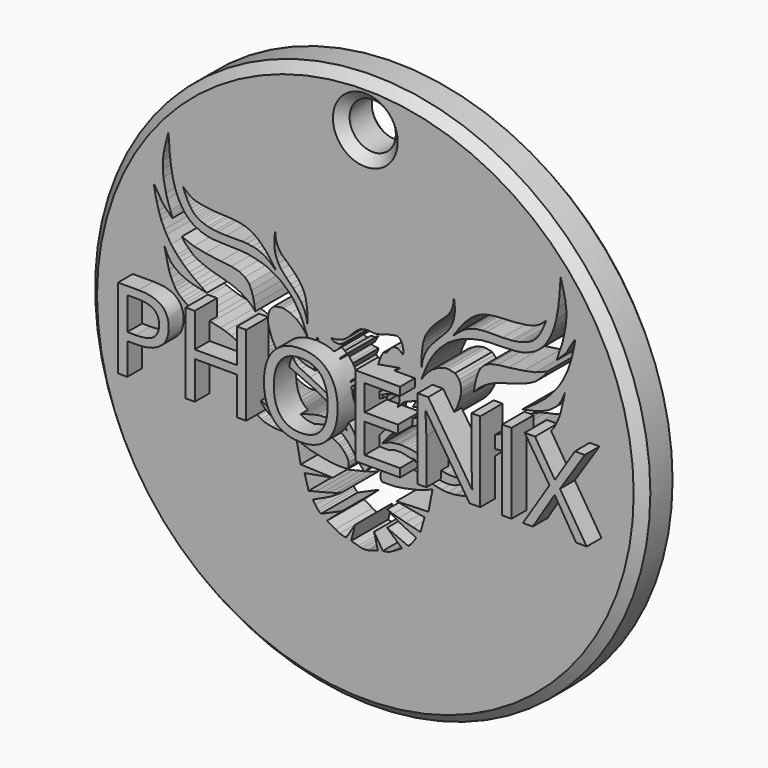
from build123d import *

# Parameters (mm, degrees)
F0_R         = 30
F1_DEPTH     = 5
F3_DEPTH     = 6
F5_START     = 4
F4_TEXT_SIZE = 12.110579539
F5_DEPTH     = 3
F6_R         = 2.5
F7_DEPTH     = 25
F8_SIZE      = 1


# Not quite as in the source:
# - Text() gives the source's letters only with a copy of the font that has no kerning and outlines rounded to 1/6400 em; it was checked with that copy


with BuildPart() as f1:
    # F0 (on Front) → F1 (new body)
    with BuildSketch(Plane.XZ):
        with Locations((-0.3908925251, -0.4964765349)):
            Circle(F0_R)
    extrude(amount=F1_DEPTH)

    # F2 (on Front) → F3 (cut)
    with BuildSketch(Plane.XZ):
        Polygon((-6.9009796716, 3.3349313308), (-6.5914276056, 2.8706034645), (-6.844074931, 3.5021796357), (-7.0858872496, 4.1097938083), (-7.3660952039, 4.7416752204), (-7.6773129404, 5.2794478834), (-7.8633381054, 5.5755167268), (-8.0336434767, 5.8401445858), (-8.2278484479, 6.1087491922), (-8.6159808561, 6.5514193848), (-9.1884760186, 7.0818513632), (-9.5344837755, 7.3751141317), (-10.111220181, 7.7330595814), (-10.5915460736, 7.9969679937), (-11.0050672665, 8.1910705194), (-11.4291384816, 8.3514153957), (-12.170586735, 8.565209806), (-13.1030725315, 8.7572177872), (-13.9272995293, 8.8297724724), (-15.3120374307, 8.863019757), (-16.7676210403, 8.9269923046), (-17.4451787025, 9.0234624222), (-18.1944258511, 9.2512723058), (-18.9065337181, 9.5856180415), (-19.2718468606, 9.8555041477), (-19.5480845869, 10.1086637005), (-19.8738295585, 10.4359621182), (-20.1065801084, 10.7434652746), (-20.4004887491, 11.2334582955), (-20.6413529813, 11.6951130331), (-20.7818560302, 12.0313186198), (-20.96250467, 12.5180631876), (-21.2009325624, 13.3876278996), (-21.4092768729, 14.5726772025), (-21.5388201177, 15.719242394), (-21.5902812779, 16.5217351168), (-21.6488484293, 17.2635931522), (-21.6683708131, 17.5434164703), (-21.8048263341, 17.0381870121), (-21.9664536417, 16.4239984006), (-22.1739932895, 15.4715124518), (-22.2793165594, 14.6293323487), (-22.2793165594, 13.8129889965), (-22.2095865756, 13.0682913586), (-21.9386145473, 11.6732902825), (-21.7981114984, 11.1614549533), (-21.4531756938, 10.173773393), (-21.377377212, 9.9247004837), (-21.3046371937, 9.7339823842), (-21.246092394, 9.5060067251), (-21.4333534241, 9.6954731271), (-21.5672496706, 9.834151715), (-21.839980036, 10.11552196), (-22.0640357584, 10.340699926), (-22.2723558545, 10.5769401416), (-22.3979391158, 10.74438449), (-22.4664080888, 10.8877671883), (-22.6057190448, 11.1188190058), (-22.8970702738, 11.6094984114), (-22.9983050376, 11.7736626416), (-23.1433175504, 12.0034934953), (-23.2253987342, 12.0978886262), (-23.2127886266, 11.8879470974), (-23.1080465019, 11.3241076469), (-22.9371320456, 10.5622867122), (-22.7170959115, 9.7489971668), (-22.5869454443, 9.3390233815), (-22.4437788129, 8.935556747), (-22.0956355333, 8.1833088771), (-21.8711271882, 7.7473041601), (-21.3806033134, 6.9752070121), (-20.7347813994, 6.1996374279), (-20.5585248768, 6.0046529397), (-20.2825926244, 5.7213520631), (-19.9078507721, 5.3766006604), (-19.4278676063, 4.9743568525), (-19.1152207553, 4.7224150039), (-18.7558140606, 4.458708223), (-18.3370038867, 4.1675912216), (-18.016314134, 3.9481716231), (-17.5145696032, 3.6100379748), (-18.3822226251, 3.7996887131), (-18.9730655402, 3.9288345724), (-19.6079221196, 4.1365632488), (-19.850788638, 4.2308908887), (-20.2664192766, 4.4228830375), (-20.6319325281, 4.6325615132), (-20.9945701038, 4.9115952627), (-21.1902355569, 5.0785678585), (-21.430300944, 5.3341447191), (-21.6075535864, 5.6020328775), (-21.7487941244, 5.8274169327), (-21.8645335297, 6.0821418594), (-22.052251676, 6.4952811086), (-22.143593058, 6.7417933606), (-21.8687430024, 5.5104247294), (-21.7532683164, 5.0212959759), (-21.5998519291, 4.4266222568), (-21.3759932667, 3.8224721793), (-21.1102589965, 3.2944113482), (-20.9858700509, 3.0643832629), (-20.816994831, 2.8091561981), (-20.5768158773, 2.5236710225), (-20.2444986021, 2.2400855596), (-19.9949573725, 2.0480745006), (-19.7460502386, 1.8908699276), (-19.3919268787, 1.7100296436), (-18.7242198735, 1.4506969601), (-18.1349273771, 1.265995088), (-17.4961388111, 1.1113942601), (-17.0138068497, 0.9861360304), (-16.0548575222, 0.776529836), (-15.4994018376, 0.6271853927), (-14.9125047028, 0.3992386919), (-14.462351799, 0.1868291292), (-14.191233553, 0.0221533028), (-13.8414734975, -0.2469717583), (-13.7188884659, -0.3515806231), (-13.5706374333, -0.4838758298), (-13.4206879884, -0.6435140385), (-13.1936527732, -0.9473082846), (-13.0392471328, -1.1806669645), (-12.9114612937, -1.4318333706), (-12.7589125186, -1.7675701529), (-12.6668820158, -1.9539315253), (-12.6758497208, -2.0026378334), (-12.9692815244, -1.8056348199), (-13.1037309766, -1.7221844755), (-13.3441239595, -1.5867486363), (-13.5315451771, -1.4814096503), (-13.7764243409, -1.3569180155), (-14.0087269247, -1.2713534525), (-14.3553037196, -1.1796122417), (-14.5744634792, -1.1303438805), (-14.9550195783, -1.0606886353), (-15.3880430592, -1.0301302617), (-15.4070062563, -1.0419205064), (-14.3769606948, -1.9611052703), (-13.950872235, -2.4897714611), (-13.8280401006, -2.6754119899), (-13.7659199536, -2.7864235453), (-13.6367864907, -3.0263995286), (-13.5693699121, -3.1559108756), (-13.4732011494, -3.3553417639), (-13.3834818983, -3.5782567641), (-13.3483398499, -3.665570129), (-13.3177542287, -3.7415626689), (-13.2900051499, -3.8164519222), (-13.2579220653, -3.8961650353), (-13.1716039032, -4.1291206144), (-13.1037309766, -4.2977565899), (-13.0368275568, -4.5038657263), (-12.9336360842, -4.755594302), (-12.8743490204, -4.9155983143), (-12.8289693967, -5.0395550206), (-12.7818249166, -5.179558415), (-12.7129619941, -5.3162728436), (-12.6529606059, -5.441990681), (-12.5875174999, -5.5690663867), (-12.5018004328, -5.717641674), (-12.4399675409, -5.8170924781), (-12.3709030449, -5.8906194754), (-12.2719677165, -6.0149733908), (-12.2122876346, -6.0785096139), (-12.1162394062, -6.1718025245), (-11.9583159685, -6.3006826676), (-11.6442255676, -6.48872694), (-11.4394053817, -6.5820780583), (-11.263766326, -6.651269272), (-10.9468530864, -6.7377560772), (-10.4531301185, -6.8261306733), (-10.1994303986, -6.8651614711), (-9.4673996791, -6.9074714556), (-8.8127674535, -6.8461140618), (-8.1605101004, -6.7201512866), (-7.7530797571, -6.601061672), (-7.6366481371, -6.5667750314), (-7.1542183869, -6.3989814371), (-6.7082373425, -6.2484969385), (-6.3224504702, -6.1034848914), (-6.0155452229, -5.9889322147), (-5.7466630824, -5.8877016418), (-5.4877381772, -5.793986842), (-5.3067770787, -5.7256827131), (-5.0938818604, -5.6618140079), (-4.9314326607, -5.6130257435), (-4.4543091208, -5.6298798881), (-4.2681246996, -5.6629236788), (-3.8872428704, -5.7842899114), (-3.6318132188, -5.9038903564), (-3.3626011573, -6.0657951981), (-3.2329140231, -6.1565763317), (-3.1198710203, -6.2322891317), (-3.0065586325, -6.325469818), (-2.8050330002, -6.5247113816), (-2.6203475427, -6.7271809094), (-2.4301900994, -6.9857402705), (-2.3060552776, -7.2086802684), (-2.1962239407, -7.4997954071), (-2.1979229059, -7.8905448318), (-2.2251054179, -7.9788882285), (-2.2998573259, -8.1215966493), (-2.3934820201, -8.2066971809), (-2.5116000324, -8.2011017948), (-3.1098364852, -8.2135656849), (-3.6893782672, -8.1886388361), (-4.1131288745, -8.13878607), (-4.7487551346, -8.0390796065), (-5.3594545461, -7.9144472256), (-6.4499899745, -7.6651819982), (-7.2787967511, -7.3722954839), (-7.8291641548, -7.1412432007), (-7.3802727275, -9.4111217186), (-3.9100204594, -9.5452908427), (-5.1035000943, -9.7587769851), (-5.6091333916, -9.8464553431), (-6.3824308752, -9.9857078539), (-6.9622276351, -10.0901154801), (-6.5257768147, -11.6362702101), (-5.7188435458, -11.4410445094), (-4.9314326607, -11.2490728498), (-4.1830670089, -11.0505931079), (-3.5453294404, -10.874889791), (-2.9302015544, -10.6291441345), (-3.2655058894, -10.8683817089), (-4.1545955464, -11.4114684984), (-4.7202953137, -11.6943186149), (-5.962850526, -12.2760608792), (-6.0480938971, -12.3117221519), (-6.0583320446, -12.3439328745), (-5.7991264497, -12.7167284), (-5.5476897396, -13.0691304803), (-5.4026274078, -13.2278686718), (-5.2478690632, -13.359698467), (-5.1814815961, -13.3798383176), (-5.1269410178, -13.3649753407), (-2.913645003, -12.3976254836), (-4.5224814676, -13.8263506815), (-3.6250384645, -14.3688376834), (-3.1727361493, -14.6062457934), (-2.6696813293, -14.7449653596), (-2.4519131985, -14.7449653596), (-1.5037892153, -13.2389152423), (-1.9168391591, -14.9040902033), (-1.1345401872, -15.122467652), (-0.889661198, -15.2004463598), (-0.6817192771, -15.2363106608), (-0.4773337569, -15.2363106608), (-0.2729482367, -15.2363106608), (-0.0650063157, -15.2004463598), (0.1798726735, -15.122467652), (0.9621716454, -14.9040902033), (0.5491217016, -13.2389152423), (1.4972456847, -14.7449653596), (1.7150138156, -14.7449653596), (2.2180686356, -14.6062457934), (2.6703709508, -14.3688376834), (3.5678139539, -13.8263506815), (1.9589774893, -12.3976254836), (4.1722735041, -13.3649753407), (4.2268140824, -13.3798383176), (4.2932015494, -13.359698467), (4.4479598941, -13.2278686718), (4.5930222259, -13.0691304803), (4.844458936, -12.7167284), (5.1036645309, -12.3439328745), (5.0934263834, -12.3117221519), (5.0081830123, -12.2760608792), (3.7656278, -11.6943186149), (3.1999280327, -11.4114684984), (2.3108383757, -10.8683817089), (1.9755340406, -10.6291441345), (2.5906619267, -10.874889791), (3.2283994951, -11.0505931079), (3.9767651469, -11.2490728498), (4.764176032, -11.4410445094), (5.5711093009, -11.6362702101), (6.0075601214, -10.0901154801), (5.4277633614, -9.9857078539), (4.6544658779, -9.8464553431), (4.1488325805, -9.7587769851), (2.9553529457, -9.5452908427), (6.4256052137, -9.4111217186), (6.8744966411, -7.1412432007), (6.3241292373, -7.3722954839), (5.4953224608, -7.6651819982), (4.4047870324, -7.9144472256), (3.7940876209, -8.0390796065), (3.1584613607, -8.13878607), (2.7347107534, -8.1886388361), (2.1551689715, -8.2135656849), (1.5569325187, -8.2011017948), (1.4388145064, -8.2066971809), (1.3451898121, -8.1215966493), (1.2704379042, -7.9788882285), (1.2432553922, -7.8905448318), (1.241556427, -7.4997954071), (1.3513877639, -7.2086802684), (1.4755225857, -6.9857402705), (1.665680029, -6.7271809094), (1.8503654865, -6.5247113816), (2.0518911188, -6.325469818), (2.1652035066, -6.2322891317), (2.2782465094, -6.1565763317), (2.4079336436, -6.0657951981), (2.6771457051, -5.9038903564), (2.9325753567, -5.7842899114), (3.3134571859, -5.6629236788), (3.499641607, -5.6298798881), (3.9767651469, -5.6130257435), (4.1392143467, -5.6618140079), (4.3521095649, -5.7256827131), (4.5330706635, -5.793986842), (4.7919955687, -5.8877016418), (5.0608777092, -5.9889322147), (5.3677829565, -6.1034848914), (5.7535698288, -6.2484969385), (6.1995508731, -6.3989814371), (6.6819806234, -6.5667750314), (6.7984122434, -6.601061672), (7.2058425867, -6.7201512866), (7.8580999398, -6.8461140618), (8.5127321654, -6.9074714556), (9.2447628849, -6.8651614711), (9.4984626048, -6.8261306733), (9.9921855726, -6.7377560772), (10.3090988123, -6.651269272), (10.484737868, -6.5820780583), (10.6895580539, -6.48872694), (11.0036484548, -6.3006826676), (11.1615718924, -6.1718025245), (11.2576201209, -6.0785096139), (11.3173002028, -6.0149733908), (11.4162355312, -5.8906194754), (11.4853000272, -5.8170924781), (11.5471329191, -5.717641674), (11.6328499862, -5.5690663867), (11.6982930922, -5.441990681), (11.7582944804, -5.3162728436), (11.8271574029, -5.179558415), (11.8743018829, -5.0395550206), (11.9196815067, -4.9155983143), (11.9789685705, -4.755594302), (12.0821600431, -4.5038657263), (12.1490634629, -4.2977565899), (12.2169363894, -4.1291206144), (12.3032545516, -3.8961650353), (12.3353376362, -3.8164519222), (12.363086715, -3.7415626689), (12.3936723362, -3.665570129), (12.4288143846, -3.5782567641), (12.5185336357, -3.3553417639), (12.6147023984, -3.1559108756), (12.682118977, -3.0263995286), (12.8112524399, -2.7864235453), (12.8733725869, -2.6754119899), (12.9962047213, -2.4897714611), (13.4222931811, -1.9611052703), (14.4523387426, -1.0419205064), (14.4333755455, -1.0301302617), (14.0003520646, -1.0606886353), (13.6197959655, -1.1303438805), (13.4006362059, -1.1796122417), (13.0540594109, -1.2713534525), (12.8217568272, -1.3569180155), (12.5768776634, -1.4814096503), (12.3894564458, -1.5867486363), (12.1490634629, -1.7221844755), (12.0146140107, -1.8056348199), (11.7211822071, -2.0026378334), (11.712214502, -1.9539315253), (11.8042450049, -1.7675701529), (11.95679378, -1.4318333706), (12.0845796191, -1.1806669645), (12.2389852594, -0.9473082846), (12.4660204747, -0.6435140385), (12.6159699196, -0.4838758298), (12.7642209522, -0.3515806231), (12.8868059837, -0.2469717583), (13.2365660393, 0.0221533028), (13.5076842853, 0.1868291292), (13.9578371891, 0.3992386919), (14.5447343239, 0.6271853927), (15.1001900085, 0.776529836), (16.059139336, 0.9861360304), (16.5414712974, 1.1113942601), (17.1802598634, 1.265995088), (17.7695523598, 1.4506969601), (18.437259365, 1.7100296436), (18.7913827249, 1.8908699276), (19.0402898588, 2.0480745006), (19.2898310884, 2.2400855596), (19.6221483636, 2.5236710225), (19.8623273172, 2.8091561981), (20.0312025372, 3.0643832629), (20.1555914828, 3.2944113482), (20.421325753, 3.8224721793), (20.6451844154, 4.4266222568), (20.7986008027, 5.0212959759), (20.9140754887, 5.5104247294), (21.1889255443, 6.7417933606), (21.0975841623, 6.4952811086), (20.909866016, 6.0821418594), (20.7941266106, 5.8274169327), (20.6528860726, 5.6020328775), (20.4756334302, 5.3341447191), (20.2355680432, 5.0785678585), (20.0399025901, 4.9115952627), (19.6772650143, 4.6325615132), (19.3117517629, 4.4228830375), (18.8961211243, 4.2308908887), (18.6532546059, 4.1365632488), (18.0183980265, 3.9288345724), (17.4275551114, 3.7996887131), (16.5599020895, 3.6100379748), (17.0616466203, 3.9481716231), (17.382336373, 4.1675912216), (17.8011465468, 4.458708223), (18.1605532416, 4.7224150039), (18.4732000926, 4.9743568525), (18.9531832584, 5.3766006604), (19.3279251107, 5.7213520631), (19.6038573631, 6.0046529397), (19.7801138856, 6.1996374279), (20.4259357997, 6.9752070121), (20.9164596745, 7.7473041601), (21.1409680196, 8.1833088771), (21.4891112992, 8.935556747), (21.6322779306, 9.3390233815), (21.7624283978, 9.7489971668), (21.9824645319, 10.5622867122), (22.1533789882, 11.3241076469), (22.2581211128, 11.8879470974), (22.2707312205, 12.0978886262), (22.1886500367, 12.0034934953), (22.0436375239, 11.7736626416), (21.94240276, 11.6094984114), (21.6510515311, 11.1188190058), (21.5117405751, 10.8877671883), (21.443271602, 10.74438449), (21.3176883408, 10.5769401416), (21.1093682447, 10.340699926), (20.8853125223, 10.11552196), (20.6125821569, 9.834151715), (20.4786859103, 9.6954731271), (20.2914248803, 9.5060067251), (20.34996968, 9.7339823842), (20.4227096983, 9.9247004837), (20.49850818, 10.173773393), (20.8434439846, 11.1614549533), (20.9839470335, 11.6732902825), (21.2549190619, 13.0682913586), (21.3246490457, 13.8129889965), (21.3246490457, 14.6293323487), (21.2193257757, 15.4715124518), (21.0117861279, 16.4239984006), (20.8501588204, 17.0381870121), (20.7137032994, 17.5434164703), (20.6941809156, 17.2635931522), (20.6356137642, 16.5217351168), (20.584152604, 15.719242394), (20.4546093591, 14.5726772025), (20.2462650486, 13.3876278996), (20.0078371563, 12.5180631876), (19.8271885165, 12.0313186198), (19.6866854676, 11.6951130331), (19.4458212354, 11.2334582955), (19.1519125947, 10.7434652746), (18.9191620448, 10.4359621182), (18.5934170731, 10.1086637005), (18.3171793469, 9.8555041477), (17.9518662044, 9.5856180415), (17.2397583374, 9.2512723058), (16.4905111887, 9.0234624222), (15.8129535266, 8.9269923046), (14.357369917, 8.863019757), (12.9726320156, 8.8297724724), (12.1484050178, 8.7572177872), (11.2159192213, 8.565209806), (10.4744709679, 8.3514153957), (10.0503997528, 8.1910705194), (9.6368785598, 7.9969679937), (9.1565526673, 7.7330595814), (8.5798162618, 7.3751141317), (8.2338085049, 7.0818513632), (7.6613133424, 6.5514193848), (7.2731809341, 6.1087491922), (7.0789759629, 5.8401445858), (6.9086705917, 5.5755167268), (6.7226454266, 5.2794478834), (6.4114276902, 4.7416752204), (6.1312197358, 4.1097938083), (5.8894074173, 3.5021796357), (5.6367600919, 2.8706034645), (5.9463121579, 3.3349313308), (6.3255131827, 3.7837815471), (6.8517514155, 4.2481096461), (7.5172880315, 4.619571846), (8.2911677309, 4.8439968377), (8.6161974468, 4.8439968377), (9.3043926754, 4.6935421415), (9.5365564921, 4.4768559746), (9.7455042996, 4.244692158), (9.8770638579, 3.8887073752), (9.9699288257, 3.4553345758), (9.9699288257, 3.1767380424), (9.8920525634, 2.6312284172), (9.7465864965, 2.1786685102), (9.5263780677, 1.5331205213), (9.2516099685, 1.0320723522), (8.9566377574, 0.5673905252), (8.4863552474, 0.0535830186), (7.900582219, -0.4137892101), (7.1590175503, -0.7752237143), (6.4922334277, -1.0494154412), (5.769364594, -1.3734601671), (5.3143613623, -1.5531850513), (4.8175803968, -1.799066551), (4.4362131157, -1.9797142595), (4.0548458346, -2.1954877302), (3.5897002096, -2.4586620791), (3.1866920763, -2.7417927049), (2.747433784, -3.0866917223), (2.4477891275, -3.3350461163), (2.3023235262, -3.4805119503), (2.1528171492, -3.642140422), (1.975025807, -3.8441759534), (1.8526418717, -3.9994004183), (1.7260537134, -4.1428669356), (1.6142340028, -4.2842240073), (1.5298179933, -4.4043259695), (1.4482704573, -4.5198518783), (1.4057977241, -4.5878081582), (1.4877891984, -4.5414182715), (1.5742309042, -4.4837985188), (1.6762433224, -4.4358973391), (1.7399483764, -4.4059838513), (1.8232696117, -4.3668593453), (1.911158617, -4.3255899871), (2.0272262045, -4.2825178243), (2.1301748347, -4.2452458292), (2.2677017234, -4.1954549626), (2.4408279569, -4.1494057514), (2.5509885163, -4.1262721643), (2.7810983011, -4.0910816751), (3.0116653652, -4.0648807772), (3.1651710742, -4.0402412415), (3.2942542466, -4.0255726458), (3.4481315524, -4.0255726458), (3.672859224, -4.0362342261), (3.9383466938, -4.0648807772), (4.3332051137, -4.0804566815), (4.6627936536, -4.1280263104), (4.8678224557, -4.179386422), (5.1014274941, -4.2290138081), (5.3231935599, -4.2778020725), (5.5955220596, -4.3665086851), (5.8127130033, -4.422603175), (5.9507582919, -4.4709192589), (6.0827513807, -4.5081526041), (6.2150448211, -4.5535927638), (6.3577858573, -4.6026214645), (6.5070544952, -4.6633598395), (6.6908556619, -4.7135576606), (6.8142712698, -4.7468063422), (6.9485898712, -4.7857123427), (7.088004204, -4.8394398764), (7.2577461251, -4.8865387216), (7.5232326635, -4.965854343), (7.8349873074, -5.0506782718), (8.0614272156, -5.0962027162), (8.4007005789, -5.1536601968), (8.6362141354, -5.1790725115), (8.9883797973, -5.1929643228), (9.1500332945, -5.1993410374), (9.3879853957, -5.1885233261), (9.5861627829, -5.1660030866), (9.7404071712, -5.1298472099), (9.8646483966, -5.096486304), (9.9701821455, -5.0710150972), (10.0580757135, -5.0332737155), (10.146530869, -4.9977004528), (10.2327583008, -4.9671088345), (10.32118086, -4.9322033301), (10.3755673044, -4.9044843763), (10.4311477044, -4.8715993762), (10.4972781264, -4.8379208893), (10.5630481266, -4.8027201556), (10.6181647279, -4.773077555), (10.7272188761, -4.7092679888), (10.8612436452, -4.630937241), (10.8412739033, -4.6890766901), (10.7994867139, -4.7463122755), (10.7605807134, -4.8018926755), (10.7114841812, -4.8639569432), (10.6834998748, -4.8993326695), (10.6483479613, -4.940148443), (10.6192342784, -4.9817397171), (10.5811642134, -5.0188680179), (10.5499748524, -5.0582953413), (10.5216738761, -5.0987255978), (10.4824812734, -5.1451963373), (10.4560577893, -5.1757604815), (10.424315522, -5.2080089226), (10.3942699613, -5.2427627365), (10.3620230802, -5.2706417628), (10.3278752067, -5.30464435), (10.2906570134, -5.3368213218), (10.2539520711, -5.3685545629), (10.2250503288, -5.3935415508), (10.1920504852, -5.4317125951), (10.1539246389, -5.4607563652), (10.1188128465, -5.4941144772), (10.072660225, -5.5309198797), (10.0375770339, -5.5612510363), (9.9701821455, -5.6091113947), (9.8752673366, -5.681604147), (9.7675598809, -5.7506351732), (9.6419132897, -5.8166729286), (9.5210248255, -5.8858408593), (9.3766633072, -5.9372195974), (9.2482562759, -5.9886099771), (9.0422849753, -6.0309884138), (8.8113700622, -6.0674720444), (8.6805193923, -6.0823414927), (8.2236533635, -6.0744425282), (7.876517775, -6.0440944508), (7.7026528888, -6.0068378225), (7.5687063509, -5.9749032371), (7.449839788, -5.9429691173), (7.3162126937, -5.9113856405), (7.2186622463, -5.8778790063), (7.1099839793, -5.8405501879), (7.0011807256, -5.8088148944), (6.8989885622, -5.7812156156), (6.7992043627, -5.7469417321), (6.7078108676, -5.7155498883), (6.6173081868, -5.681604147), (6.5443598493, -5.6565478471), (6.2595690251, -5.5642165244), (6.050497066, -5.4857978236), (5.9126201668, -5.4270457476), (5.7355196349, -5.3662152451), (5.5283531555, -5.2950576889), (5.4023499567, -5.247796415), (5.233107195, -5.1843168477), (5.0934263834, -5.1319253754), (4.7176834778, -5.0201960839), (4.4350657263, -4.9349451438), (4.1215951205, -4.8514972441), (3.9056805545, -4.8074326478), (3.6181607866, -4.7556571662), (3.4137676121, -4.7261123545), (2.8963673976, -4.7377943993), (2.6766451192, -4.7677042894), (2.5522632641, -4.8040081747), (2.4297296186, -4.8391465098), (2.25637533, -4.9019595608), (2.1061509033, -4.9714832567), (1.9376422861, -5.0599314272), (1.8782152911, -5.0963833928), (1.8337511574, -5.1278788596), (1.7962344573, -5.1598371938), (1.7559386906, -5.1908697933), (1.7258327571, -5.216807127), (1.6683999565, -5.2557131276), (1.437621715, -5.4778917693), (1.3749260106, -5.5469144136), (1.2129531824, -5.7292617857), (1.1593802483, -5.7899774984), (0.8737010066, -6.1430511996), (0.716559065, -6.3632940874), (0.6120984127, -6.5097013132), (0.49046817, -6.6939559765), (0.2669849782, -6.9867535494), (0.020992758, -7.3315248841), (-0.2362576779, -7.6294653118), (-0.4773337569, -7.8736385331), (-0.7184098358, -7.6294653118), (-0.9756602718, -7.3315248841), (-1.2216524919, -6.9867535494), (-1.4451356838, -6.6939559765), (-1.5667659264, -6.5097013132), (-1.6712265788, -6.3632940874), (-1.8283685204, -6.1430511996), (-2.114047762, -5.7899774984), (-2.1676206961, -5.7292617857), (-2.3295935243, -5.5469144136), (-2.3922892287, -5.4778917693), (-2.6230674703, -5.2557131276), (-2.6805002708, -5.216807127), (-2.7106062043, -5.1908697933), (-2.750901971, -5.1598371938), (-2.7884186711, -5.1278788596), (-2.8328828048, -5.0963833928), (-2.8923097998, -5.0599314272), (-3.060818417, -4.9714832567), (-3.2110428438, -4.9019595608), (-3.3843971323, -4.8391465098), (-3.5069307778, -4.8040081747), (-3.6313126329, -4.7677042894), (-3.8510349113, -4.7377943993), (-4.3684351258, -4.7261123545), (-4.5728283003, -4.7556571662), (-4.8603480682, -4.8074326478), (-5.0762626342, -4.8514972441), (-5.38973324, -4.9349451438), (-5.6723509915, -5.0201960839), (-6.0480938971, -5.1319253754), (-6.1877747088, -5.1843168477), (-6.3570174704, -5.247796415), (-6.4830206692, -5.2950576889), (-6.6901871486, -5.3662152451), (-6.8672876805, -5.4270457476), (-7.0051645798, -5.4857978236), (-7.2142365389, -5.5642165244), (-7.499027363, -5.6565478471), (-7.5719757006, -5.681604147), (-7.6624783814, -5.7155498883), (-7.7538718764, -5.7469417321), (-7.8536560759, -5.7812156156), (-7.9558482394, -5.8088148944), (-8.0646514931, -5.8405501879), (-8.1733297601, -5.8778790063), (-8.2708802074, -5.9113856405), (-8.4045073017, -5.9429691173), (-8.5233738646, -5.9749032371), (-8.6573204026, -6.0068378225), (-8.8311852887, -6.0440944508), (-9.1783208773, -6.0744425282), (-9.635186906, -6.0823414927), (-9.7660375759, -6.0674720444), (-9.996952489, -6.0309884138), (-10.2029237896, -5.9886099771), (-10.3313308209, -5.9372195974), (-10.4756923392, -5.8858408593), (-10.5965808034, -5.8166729286), (-10.7222273946, -5.7506351732), (-10.8299348503, -5.681604147), (-10.9248496592, -5.6091113947), (-10.9922445476, -5.5612510363), (-11.0273277387, -5.5309198797), (-11.0734803602, -5.4941144772), (-11.1085921526, -5.4607563652), (-11.1467179989, -5.4317125951), (-11.1797178425, -5.3935415508), (-11.2086195848, -5.3685545629), (-11.2453245272, -5.3368213218), (-11.2825427204, -5.30464435), (-11.316690594, -5.2706417628), (-11.3489374751, -5.2427627365), (-11.3789830357, -5.2080089226), (-11.410725303, -5.1757604815), (-11.4371487871, -5.1451963373), (-11.4763413898, -5.0987255978), (-11.5046423661, -5.0582953413), (-11.5358317271, -5.0188680179), (-11.5739017921, -4.9817397171), (-11.603015475, -4.940148443), (-11.6381673885, -4.8993326695), (-11.666151695, -4.8639569432), (-11.7152482271, -4.8018926755), (-11.7541542277, -4.7463122755), (-11.7959414171, -4.6890766901), (-11.8159111589, -4.630937241), (-11.6818863899, -4.7092679888), (-11.5728322417, -4.773077555), (-11.5177156404, -4.8027201556), (-11.4519456401, -4.8379208893), (-11.3858152181, -4.8715993762), (-11.3302348182, -4.9044843763), (-11.2758483738, -4.9322033301), (-11.1874258146, -4.9671088345), (-11.1011983827, -4.9977004528), (-11.0127432272, -5.0332737155), (-10.9248496592, -5.0710150972), (-10.8193159103, -5.096486304), (-10.6950746849, -5.1298472099), (-10.5408302966, -5.1660030866), (-10.3426529095, -5.1885233261), (-10.1047008082, -5.1993410374), (-9.943047311, -5.1929643228), (-9.5908816491, -5.1790725115), (-9.3553680927, -5.1536601968), (-9.0160947293, -5.0962027162), (-8.7896548212, -5.0506782718), (-8.4779001772, -4.965854343), (-8.2124136388, -4.8865387216), (-8.0426717177, -4.8394398764), (-7.9032573849, -4.7857123427), (-7.7689387836, -4.7468063422), (-7.6455231756, -4.7135576606), (-7.4617220089, -4.6633598395), (-7.312453371, -4.6026214645), (-7.1697123349, -4.5535927638), (-7.0374188945, -4.5081526041), (-6.9054258056, -4.4709192589), (-6.767380517, -4.422603175), (-6.5501895733, -4.3665086851), (-6.2778610736, -4.2778020725), (-6.0560950078, -4.2290138081), (-5.8224899694, -4.179386422), (-5.6174611673, -4.1280263104), (-5.2878726274, -4.0804566815), (-4.8930142075, -4.0648807772), (-4.6275267377, -4.0362342261), (-4.4027990662, -4.0255726458), (-4.2489217603, -4.0255726458), (-4.1198385879, -4.0402412415), (-3.9663328789, -4.0648807772), (-3.7357658148, -4.0910816751), (-3.50565603, -4.1262721643), (-3.3954954706, -4.1494057514), (-3.2223692371, -4.1954549626), (-3.0848423485, -4.2452458292), (-2.9818937182, -4.2825178243), (-2.8658261307, -4.3255899871), (-2.7779371254, -4.3668593453), (-2.6946158901, -4.4059838513), (-2.6309108362, -4.4358973391), (-2.5288984179, -4.4837985188), (-2.4424567121, -4.5414182715), (-2.3604652379, -4.5878081582), (-2.4029379711, -4.5198518783), (-2.484485507, -4.4043259695), (-2.5689015165, -4.2842240073), (-2.6807212271, -4.1428669356), (-2.8073093854, -3.9994004183), (-2.9296933208, -3.8441759534), (-3.1074846629, -3.642140422), (-3.25699104, -3.4805119503), (-3.4024566412, -3.3350461163), (-3.7021012977, -3.0866917223), (-4.14135959, -2.7417927049), (-4.5443677234, -2.4586620791), (-5.0095133483, -2.1954877302), (-5.3908806294, -1.9797142595), (-5.7722479105, -1.799066551), (-6.269028876, -1.5531850513), (-6.7240321077, -1.3734601671), (-7.4469009414, -1.0494154412), (-8.113685064, -0.7752237143), (-8.8552497327, -0.4137892101), (-9.4410227612, 0.0535830186), (-9.9113052711, 0.5673905252), (-10.2062774822, 1.0320723522), (-10.4810455814, 1.5331205213), (-10.7012540102, 2.1786685102), (-10.8467200771, 2.6312284172), (-10.9245963395, 3.1767380424), (-10.9245963395, 3.4553345758), (-10.8317313716, 3.8887073752), (-10.7001718134, 4.244692158), (-10.4912240058, 4.4768559746), (-10.2590601891, 4.6935421415), (-9.5708649606, 4.8439968377), (-9.2458352447, 4.8439968377), (-8.4719555452, 4.619571846), (-7.8064189292, 4.2481096461), (-7.2801806964, 3.7837815471), align=None)
        Polygon((-12.3781235889, 4.1850856505), (-12.2784171253, 3.5556911025), (-12.5446775928, 3.8274233229), (-12.8250261769, 4.1156318039), (-13.2583333179, 4.4581373222), (-13.5570224375, 4.6467827633), (-13.8661917299, 4.8301881179), (-14.3168447539, 5.0528948195), (-14.9279991165, 5.2887541242), (-15.6108802184, 5.4907896556), (-16.2089057267, 5.6604994461), (-16.8028902262, 5.8261686936), (-17.3807181418, 6.0100448318), (-17.8825184703, 6.2007284723), (-18.4043888003, 6.4315563068), (-18.9833811737, 6.7602685147), (-19.4298220614, 7.1739078585), (-19.8796782643, 7.5907115825), (-20.2259197831, 8.09752848), (-18.9274763565, 7.6029663039), (-17.678912729, 7.3458747938), (-16.0275306553, 7.1153044701), (-14.8707749322, 6.9893188775), (-14.0108102933, 6.7961383611), (-13.4001104161, 6.4658620395), (-12.9389697686, 5.9673315845), (-12.7021679655, 5.4251798429), (-12.5214513391, 4.8581017181), align=None, mode=Mode.SUBTRACT)
        Polygon((11.5900100791, 3.8274233229), (11.3237496116, 3.5556911025), (11.4234560751, 4.1850856505), (11.5667838254, 4.8581017181), (11.7475004517, 5.4251798429), (11.9843022549, 5.9673315845), (12.4454429024, 6.4658620395), (13.0561427795, 6.7961383611), (13.9161074185, 6.9893188775), (15.0728631415, 7.1153044701), (16.7242452153, 7.3458747938), (17.9728088428, 7.6029663039), (19.2712522694, 8.09752848), (18.9250107505, 7.5907115825), (18.4751545477, 7.1739078585), (18.02871366, 6.7602685147), (17.4497212865, 6.4315563068), (16.9278509566, 6.2007284723), (16.4260506281, 6.0100448318), (15.8482227125, 5.8261686936), (15.2542382129, 5.6604994461), (14.6562127047, 5.4907896556), (13.9733316028, 5.2887541242), (13.3621772402, 5.0528948195), (12.9115242162, 4.8301881179), (12.6023549237, 4.6467827633), (12.3036658042, 4.4581373222), (11.8703586631, 4.1156318039), align=None, mode=Mode.SUBTRACT)
        Polygon((-6.7403768189, 4.7225398012), (-6.6219759174, 3.8750381209), (-6.6281920299, 4.7691878863), (-6.6573456861, 5.2999174222), (-6.6931368783, 5.661085248), (-6.7515973933, 6.0929879546), (-6.8106721155, 6.46431325), (-6.9105871953, 6.8414509296), (-7.009126246, 7.1072075516), (-7.1427500807, 7.3901759461), (-7.27649685, 7.6121599413), (-7.4199633673, 7.8315790743), (-7.6098460704, 8.1100733951), (-7.7495765872, 8.2709230483), (-7.8959567472, 8.4460321814), (-8.1216832623, 8.675863035), (-8.3837518468, 8.9373420924), (-8.6458576843, 9.1841565445), (-8.9202681556, 9.435903281), (-9.2752892524, 9.7673395649), (-9.4953756779, 9.9900467321), (-9.7783440724, 10.3882979602), (-9.9119683728, 10.6869870797), (-10.0190220401, 10.9882745892), (-10.0805833936, 11.2947151065), (-10.1243611425, 11.825514026), (-10.163561441, 11.6704311222), (-10.2221295238, 11.1799947917), (-10.2367252111, 10.5233946815), (-10.1587567478, 9.9621098489), (-10.1059880108, 9.7302608192), (-10.0083751604, 9.421152994), (-9.7924163565, 8.9331166819), (-9.4813015312, 8.4664430469), (-8.9107491076, 7.8312633559), (-8.4733245894, 7.391193416), (-8.1804860383, 7.0918472484), (-7.8122168779, 6.6855028272), (-7.6003419235, 6.4424695447), (-7.3012234643, 6.0187187046), (-6.9647156633, 5.3893239237), align=None)
        Polygon((-19.9279990047, 12.7332331613), (-20.1001372188, 12.9033457488), (-19.9717544019, 12.5784557313), (-19.8933016509, 12.3688494787), (-19.7858735919, 12.1344421059), (-19.6791663766, 11.8868267164), (-19.5237044245, 11.5761058405), (-19.3886775523, 11.3587956876), (-19.2234478891, 11.1027453095), (-19.0194379538, 10.840636678), (-18.8443288207, 10.6682637706), (-18.6833851039, 10.5321649462), (-18.5511913151, 10.4451375082), (-18.4145923704, 10.3702284396), (-18.254859373, 10.2854045108), (-18.029646948, 10.183583945), (-17.8093258291, 10.0998617709), (-17.4207426608, 9.9732270464), (-17.1717796475, 9.9247554317), (-16.6344325989, 9.8331542686), (-16.3470245898, 9.8012201488), (-15.404692851, 9.7544956952), (-13.6874429882, 9.7544956952), (-13.2289286703, 9.7243394703), (-12.5572374091, 9.6347499639), (-12.1437152848, 9.5292590559), (-11.7723895237, 9.398451075), (-11.4320619032, 9.2540187761), (-11.1456084996, 9.0814046562), (-10.9469061717, 8.9421356097), (-10.7141090557, 8.7643442675), (-10.5912489817, 8.660055697), (-10.3811817244, 8.4837535396), (-10.062282905, 8.1926519051), (-10.1110721007, 8.3008734509), (-10.2973552421, 8.5492515936), (-10.5252340436, 8.8474582881), (-10.7494900003, 9.1787455603), (-10.8986739069, 9.371669963), (-11.0628381371, 9.5796119422), (-11.20785065, 9.7492486238), (-11.4512527362, 10.0076971576), (-11.6277290508, 10.1882787421), (-11.8681695312, 10.4132089764), (-12.0958229527, 10.6085836887), (-12.3030906543, 10.7580879703), (-12.6246763393, 10.9605798498), (-13.026656583, 11.1602656543), (-13.3375572041, 11.2825874239), (-13.7908384204, 11.4021757618), (-14.1095910221, 11.4623690024), (-14.6494554356, 11.5364016965), (-15.5513519421, 11.5952147171), (-16.6210234165, 11.6395205259), (-17.8603939712, 11.7796519771), (-18.7063720077, 11.9618633762), (-18.968174234, 12.0756216347), (-19.324503839, 12.2642675415), (-19.6074731648, 12.4738737941), align=None)
        Polygon((5.7384693646, 5.661085248), (5.7026781724, 5.2999174222), (5.6735245162, 4.7691878863), (5.6673084036, 3.8750381209), (5.7857093052, 4.7225398012), (6.0100481496, 5.3893239237), (6.3465559506, 6.0187187046), (6.6456744098, 6.4424695447), (6.8575493642, 6.6855028272), (7.2258185246, 7.0918472484), (7.5186570757, 7.391193416), (7.9560815939, 7.8312633559), (8.5266340175, 8.4664430469), (8.8377488428, 8.9331166819), (9.0537076467, 9.421152994), (9.151320497, 9.7302608192), (9.2040892341, 9.9621098489), (9.2820576974, 10.5233946815), (9.26746201, 11.1799947917), (9.2088939273, 11.6704311222), (9.1696936288, 11.825514026), (9.1259158798, 11.2947151065), (9.0643545263, 10.9882745892), (8.957300859, 10.6869870797), (8.8236765587, 10.3882979602), (8.5407081642, 9.9900467321), (8.3206217387, 9.7673395649), (7.9656006419, 9.435903281), (7.6911901706, 9.1841565445), (7.4290843331, 8.9373420924), (7.1670157486, 8.675863035), (6.9412892335, 8.4460321814), (6.7949090735, 8.2709230483), (6.6551785567, 8.1100733951), (6.4652958536, 7.8315790743), (6.3218293362, 7.6121599413), (6.188082567, 7.3901759461), (6.0544587323, 7.1072075516), (5.9559196816, 6.8414509296), (5.8560046018, 6.46431325), (5.7969298796, 6.0929879546), align=None)
        Polygon((11.141155439, 10.6085836887), (10.9135020175, 10.4132089764), (10.6730615371, 10.1882787421), (10.4965852224, 10.0076971576), (10.2531831362, 9.7492486238), (10.1081706234, 9.5796119422), (9.9440063932, 9.371669963), (9.7948224866, 9.1787455603), (9.5705665299, 8.8474582881), (9.3426877283, 8.5492515936), (9.156404587, 8.3008734509), (9.1076153913, 8.1926519051), (9.4265142106, 8.4837535396), (9.6365814679, 8.660055697), (9.759441542, 8.7643442675), (9.992238658, 8.9421356097), (10.1909409859, 9.0814046562), (10.4773943895, 9.2540187761), (10.81772201, 9.398451075), (11.189047771, 9.5292590559), (11.6025698953, 9.6347499639), (12.2742611566, 9.7243394703), (12.7327754744, 9.7544956952), (14.4500253373, 9.7544956952), (15.3923570761, 9.8012201488), (15.6797650852, 9.8331542686), (16.2171121337, 9.9247554317), (16.466075147, 9.9732270464), (16.8546583154, 10.0998617709), (17.0749794343, 10.183583945), (17.3001918592, 10.2854045108), (17.4599248567, 10.3702284396), (17.5965238013, 10.4451375082), (17.7287175902, 10.5321649462), (17.889661307, 10.6682637706), (18.0647704401, 10.840636678), (18.2687803754, 11.1027453095), (18.4340100386, 11.3587956876), (18.5690369108, 11.5761058405), (18.7244988629, 11.8868267164), (18.8312060782, 12.1344421059), (18.9386341372, 12.3688494787), (19.0170868882, 12.5784557313), (19.1454697051, 12.9033457488), (18.973331491, 12.7332331613), (18.6528056511, 12.4738737941), (18.3698363253, 12.2642675415), (18.0135067203, 12.0756216347), (17.751704494, 11.9618633762), (16.9057264575, 11.7796519771), (15.6663559028, 11.6395205259), (14.5966844284, 11.5952147171), (13.6947879218, 11.5364016965), (13.1549235084, 11.4623690024), (12.8361709067, 11.4021757618), (12.3828896903, 11.2825874239), (12.0719890692, 11.1602656543), (11.6700088256, 10.9605798498), (11.3484231406, 10.7580879703), align=None)
        Polygon((-1.0744505562, -5.4274941795), (-0.5022944039, -6.579538118), (-0.469290273, -6.589693483), (-0.1317237038, -5.9062326327), (0.0188159156, -5.640279036), (0.1593196794, -5.3592715412), (0.5042702542, -4.7736475244), (0.7652057684, -4.3722083792), (1.1955550872, -3.7756867241), (1.4591099462, -3.4763403237), (1.6640970716, -3.2290543895), (1.9986375701, -2.8834785335), (2.2410801612, -2.6491172612), (2.7794162743, -2.2398196161), (3.2238946296, -1.9206034485), (3.8138385862, -1.5609801048), (4.5712026767, -1.1773512233), (5.0851944834, -0.9257459897), (5.7413438335, -0.6219341303), (6.2751243822, -0.3518791054), (6.7012947984, -0.1104240218), (6.8629235029, 0.026960146), (6.9801039062, 0.1481815125), (7.0932437666, 0.3178913903), (7.1780988947, 0.5037641386), (7.2508319281, 0.9159166948), (7.2387093678, 1.2553364504), (7.2023430839, 1.5018198173), (7.1376916021, 1.659407746), (6.9946525618, 1.2596900342), (6.8289833143, 0.928351772), (6.6350293346, 0.6616647588), (6.4249122515, 0.4838734458), (6.0073970817, 0.3272694885), (5.6209964678, 0.2053840872), (5.226931069, 0.1084187461), (5.049191881, 0.0755763394), (4.8884442076, 0.0341772975), (4.7444798984, 0.0241072667), (4.7948700376, 0.1237587858), (4.9557909369, 0.4139115626), (5.0267563201, 0.5522934953), (5.0835283473, 0.6729341112), (4.9274051562, 0.6117267185), (4.5823701657, 0.4907581606), (4.1962410323, 0.3486004716), (3.9951396175, 0.2610459633), (3.758756211, 0.1147373041), (3.4971241839, -0.1061209914), (3.262674436, -0.3541618353), (3.0723966192, -0.5750201526), (3.1845245976, -0.2454316127), (3.2796636224, 0.0399852725), (3.3048666082, 0.24033316), (3.282780759, 0.3983317874), (3.1944373623, 0.5138576962), (2.9650845099, 0.5614271504), (2.6694743428, 0.5291478592), (2.1867577452, 0.4019647313), (1.7943340354, 0.2563882153), (1.307360013, 0.0692994145), (1.6322495649, -0.121966259), (1.4671847457, -0.2241492766), (1.1711160187, -0.3394326486), (0.7964449469, -0.3918342118), (0.332691212, -0.3289523593), (0.3822579747, -1.0048209224), (0.4074897734, -1.6476663295), (0.1812099072, -1.3486536918), (0.0558917709, -1.163119683), (-0.0846119365, -1.0025440715), (-0.0444680118, -1.6247746535), (0.0505218741, -2.6939781383), (0.0323325439, -3.1769871712), (-0.0106301204, -3.4744208679), (-0.1234939991, -4.0004816838), (-0.3095194988, -4.671221599), (-0.4860067274, -5.2397781983), (-0.4860067274, -4.3681971729), (-0.5022755358, -3.8280724548), (-0.5650775274, -3.366220044), (-0.6880853325, -2.8827278875), (-0.8588279597, -2.3320445325), (-1.0902949143, -1.7658121651), (-1.2224877719, -1.2678859057), (-1.2533327099, -1.2194151059), (-1.4472155599, -1.8230957212), (-1.6317070695, -1.3931822032), (-1.7297500744, -1.1298981262), (-1.7733543646, -0.8467558073), (-1.7813590821, -0.6202445948), (-1.7560221022, -0.4528003628), (-1.866182778, -0.5012710462), (-2.287841402, -0.5899044918), (-3.0248165131, -0.6537977024), (-2.6794907171, -0.262867834), (-2.5645755231, -0.1438484469), (-2.6835948229, -0.1465845271), (-2.9914036859, -0.1192237469), (-3.2195327803, -0.0254766401), (-3.3871878404, 0.0703262194), (-3.5991410259, 0.2695729199), (-3.742785193, 0.402272708), (-3.9001095574, 0.5144519382), (-4.1135237552, 0.6197909242), (-4.2845285498, 0.6156868185), (-4.3423962779, 0.535934465), (-4.318207968, 0.3297120857), (-4.2316070758, 0.0224321138), (-4.1386387311, -0.3200567735), (-4.0675010532, -0.6169212284), (-4.2689251713, -0.3745236609), (-4.4936528429, -0.1387797965), (-4.7236992978, 0.0627081099), (-4.9070166424, 0.1954078907), (-5.1532639191, 0.324003573), (-5.6613404304, 0.5029894528), (-5.9609413147, 0.6206408143), (-6.0909050517, 0.6397933466), (-6.0118483379, 0.4886985407), (-5.9217130765, 0.3425922478), (-5.8537567966, 0.1811958064), (-5.7738828473, 0.0207581343), (-6.7171351984, 0.2261065674), (-7.2985040024, 0.4213463399), (-7.5293025002, 0.5447994918), (-7.6738935895, 0.6885037874), (-7.8070457093, 0.8591119549), (-7.9356413335, 1.0848384118), (-8.0943340436, 1.4432646567), (-8.1928325817, 1.6648869496), (-8.2828393206, 1.2123066699), (-8.2659609616, 0.8135535754), (-8.2340501249, 0.6522864569), (-8.2002924755, 0.5151491496), (-8.1137912348, 0.3147177049), (-8.006574586, 0.1622326963), (-7.7618369833, -0.0867242343), (-7.3626232333, -0.3275633499), (-6.3780257478, -0.7949356223), (-4.4995676726, -1.7459092196), (-3.2149623148, -2.6591832284), (-2.3745684884, -3.485056106), (-1.693554339, -4.3750177138), align=None)
        Polygon((-0.3481850144, -3.4125503153), (-0.3059889423, -3.7205817644), (-0.1934317988, -3.2352998387), (-0.1779541344, -2.7400166728), (-0.2243869531, -1.93518179), (-0.2862973488, -1.4012047322), (-0.3327301238, -0.7047130493), (-0.3714241029, -0.4106387496), (-0.3636853071, -0.2403850958), (-0.0479175433, -0.6610153359), (0.1538284123, -0.9204029338), (0.1564484846, -0.721277087), (0.089664929, -0.0830666104), (0.1027237158, 0.0445658479), (0.2792493615, -0.0627688423), (0.4443590296, -0.0972438065), (0.8111697971, -0.1339249138), (1.1150988284, -0.1024839512), (0.6226266269, 0.2355689358), (1.0082791559, 0.2933318901), (1.3309276272, 0.4214452462), (1.6241780249, 0.6381955463), (1.4460127568, 0.879242667), (1.3242419809, 1.1833151802), (1.3041700004, 1.4291967964), (1.3944938546, 1.6650422476), (1.5450335341, 1.9109236309), (1.8059689319, 2.1618232131), (2.2339040879, 2.5204601698), (2.4542254396, 2.6570595801), (2.778532682, 2.8472086415), (3.0477663968, 3.0113719404), (3.1771054491, 3.0973115936), (3.341270145, 3.2327473164), (3.2968893647, 3.242474515), (0.9911864763, 2.8436502907), (1.1282822816, 3.2549379393), (1.3662672136, 3.8487720303), (1.4783953084, 4.0356521495), (1.5650397399, 4.1545759887), (1.6957173357, 4.2156507261), (1.8114345148, 4.2299367487), (1.9121513469, 4.2577944696), (2.0095955115, 4.3510375544), (2.1261260845, 4.512979649), (2.2859903984, 4.7273635864), (2.4117098656, 4.8666740768), (2.5748051703, 4.97200666), (2.7599863242, 5.0501567312), (3.0640913174, 5.0433608703), (3.1892559491, 4.9982657656), (3.3790876623, 4.8927050084), (3.5325495992, 4.74456558), (3.6872234195, 4.5872647315), (3.7145842798, 4.9292743206), (3.696054453, 5.243184045), (3.5997638479, 5.5949799716), (3.5106812138, 5.8045862243), (3.3901578281, 5.9853717685), (3.2539137173, 6.1111352406), (3.087145742, 6.1858971603), (2.8833078686, 6.1995773576), (2.668525558, 6.1571681872), (2.2899273317, 6.0681896284), (1.8823895371, 5.9923725203), (1.3486089883, 5.8024898171), (0.9350872715, 5.6927800179), (0.5332360743, 5.6503806263), (0.0191413747, 5.7154558599), (-0.4103553947, 5.7024406269), (-0.9049274377, 5.5722901598), (-1.2823640136, 5.3217504174), (-1.7411841545, 4.8939730041), (-2.1577766165, 4.4606663287), (-2.5036642328, 4.1579226963), (-2.8893169947, 3.9268713444), (-3.3467526082, 3.7667418364), (-3.7324051373, 3.7089788821), (-4.0789828636, 3.6851940677), (-3.9770482108, 3.5543781705), (-3.8496300112, 3.4643358085), (-3.6712444853, 3.4065728541), (-3.2923875842, 3.3997772262), (-2.9916805215, 3.4813249949), (-2.8217895888, 3.5696681589), (-2.7555320412, 3.5560769029), (-2.93154479, 3.332357388), (-3.1827646308, 3.0422550626), (-3.4338312689, 2.7827492449), (-3.6743490491, 2.5886471849), (-3.9921109565, 2.426445717), (-4.2537264526, 2.3631516378), (-4.622942768, 2.3905790877), (-4.9035465345, 2.4517634884), (-5.1356251352, 2.5783516467), (-5.2833114751, 2.7133792173), (-5.3930212744, 2.865285147), (-5.4731937125, 3.0509480275), (-5.5660251528, 3.3125637565), (-5.6377584115, 3.1353400555), (-5.6632705964, 2.8577463236), (-5.631829612, 2.5459569879), (-5.4035475478, 2.1588467062), (-5.1395231858, 1.8732862081), (-4.9052522518, 1.713851816), (-4.6709813178, 1.6422690824), (-4.5505920425, 1.6520302743), (-4.6774884686, 1.8895550165), (-4.3817725964, 1.7201043665), (-4.0661576204, 1.6875667498), (-3.7570500281, 1.7396269832), (-3.5357940942, 1.8404936418), (-3.7700650282, 1.9869129173), (-3.4186586272, 1.9869129173), (-3.1420886517, 2.0910333842), (-2.9631315265, 2.2341990843), (-3.1811338849, 1.8307323335), (-3.3763595857, 1.5313861659), (-3.5748390947, 1.3979817741), (-3.965290729, 1.245054882), (-3.649675753, 1.1506957235), (-3.3242993522, 1.0758591816), (-2.9480936937, 1.049641869), (-3.0215454753, 0.8301798371), (-3.1561953947, 0.5186540075), (-3.2321484759, 0.3836265241), (-3.0267063994, 0.2112080692), (-2.8115063906, 0.1268158958), (-2.5052193087, 0.1183190252), (-2.1549917292, 0.2216994471), (-1.8427406903, 0.3208602429), (-2.0865593106, 0.0664712352), (-2.2647245787, -0.1509951981), (-2.4428898469, -0.3579813056), (-1.99223659, -0.2872392361), (-1.6830672976, -0.0959735844), (-1.5101422323, 0.0717113871), (-1.5594252618, -0.4523040843), (-1.5594252618, -0.9630572167), (-1.4855820918, -1.174037694), (-1.4433860779, -1.1170729995), (-1.3505546376, -0.8660062449), (-1.2809310574, -0.6465865299), (-1.1965389131, -0.3765315632), (-1.1480133981, -0.5832923925), (-1.0946543189, -0.9154576692), (-1.0109896539, -1.2617626926), (-0.9219156927, -1.5581644839), (-0.8283700445, -1.8614757573), (-0.7207700401, -2.1230916027), (-0.5962915602, -2.4437818211), (-0.4895419697, -2.7711696457), (-0.4051497381, -3.0792010948), align=None)
    extrude(amount=F3_DEPTH, mode=Mode.SUBTRACT)

    # F4 (on Front) → F5 (join)
    with BuildSketch(Plane.XZ.offset(F5_START)):
        with Locations((-26.7113056034, -5.8352284832)):
            Text('PHOENIX', F4_TEXT_SIZE, font='Open Sans', text_align=(TextAlign.LEFT, TextAlign.BOTTOM))
    extrude(amount=F5_DEPTH)

    # F6 (on Front) → F7 (cut)
    with BuildSketch(Plane.XZ):
        with Locations((-0.3969778481, 24.6764719486)):
            Circle(F6_R)
    extrude(amount=F7_DEPTH, mode=Mode.SUBTRACT)

    # F8
    f8_edges = [f1.edges().sort_by_distance(p)[0] for p in [
        (-30.390893, 0, -0.496477),
        (-30.390893, -5, -0.496477),
        (-2.896978, -5, 24.676472),
        (-2.896978, 0, 24.676472),
    ]]
    chamfer(f8_edges, length=F8_SIZE)


solid = f1.part
